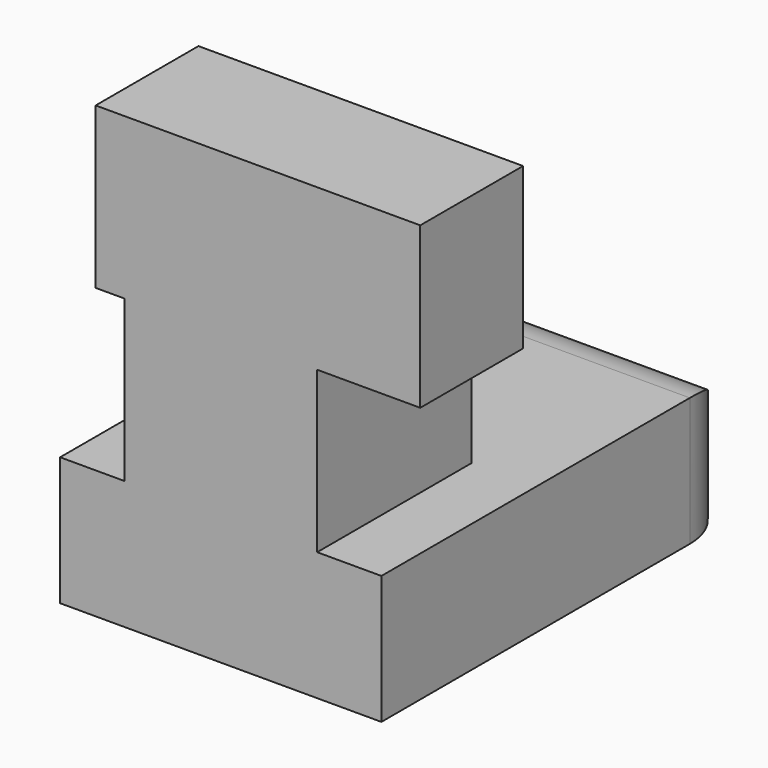
from build123d import *

# Parameters (mm, degrees)
F0_W        = 70
F0_H        = 20
F1_DEPTH    = 25
F2_W        = 30
F2_H        = 30
F3_DEPTH    = 25
F4_R        = 10
F5_W        = 50.5173448473
F5_H        = 20
F6_DEPTH    = 25
F7_T        = 2.5
F7_T3_DEPTH = 35
F7_T5_DEPTH = 35
F7_T7_DEPTH = 25


# Not quite as in the source:
# - a shell that OpenCascade refuses in one call is made with other operations: the cavity is built on its own and cut out


with BuildPart() as f1:
    # F0 (on Right) → F1 (new body, symmetric)
    with BuildSketch(Plane.YZ):
        with Locations((35, 10)):
            Rectangle(F0_W, F0_H)
    extrude(amount=F1_DEPTH, both=True)

    # F2 (on face) → F3 (join)
    with BuildSketch(Plane.XY.offset(20)):
        with Locations((0, 15)):
            Rectangle(F2_W, F2_H)
    extrude(amount=F3_DEPTH)

    # F4
    f4_edges = [f1.edges().sort_by_distance(p)[0] for p in [
        (-25, 70, 10),
        (0, 70, 20),
        (25, 70, 10),
    ]]
    fillet(f4_edges, radius=F4_R)

    # F5 (on face) → F6 (join)
    with BuildSketch(Plane.XY.offset(45)):
        with Locations((5.7856766507, 10)):
            Rectangle(F5_W, F5_H)
    extrude(amount=F6_DEPTH)

    # F7: shell of thickness 2.5, made by hand


with BuildPart() as f7_core1:
    # F7_t2: copy of F1
    add(f1.part)

    # the walls: a layer under each face that stays
    f7_faces = [f7_core1.faces().sort_by_distance(p)[0] for p in [
        (-16.6666666667, 50, 20),
        (25, 30, 10),
        (0, 67.0710678119, 17.0710678119),
        (3.0221745372, 0, 35),
        (-25, 30, 10),
        (15, 15, 32.5),
        (0, 30, 32.5),
        (-15, 15, 32.5),
        (22.0710678119, 67.0710678119, 10),
        (0, 35, 0),
        (0, 70, 5),
        (-22.0710678119, 67.0710678119, 10),
        (23.0221745372, 10, 45),
        (0, 25, 45),
        (-17.2364978865, 10, 45),
        (-19.472995773, 10, 57.5),
        (31.0443490744, 10, 57.5),
        (5.7856766507, 10, 70),
    ]]
    thicken(f7_faces, amount=-F7_T, mode=Mode.SUBTRACT)

    # F7_s4 → F7_t3 (cut)
    with BuildSketch(Plane.XZ.offset(-32.5)):
        Polygon((15.025, 20.025), (15, 17.5), (12.5, 17.5), (12.5, 20), align=None)
        Polygon((-15.025, 20.025), (-15, 17.5), (-12.5, 17.5), (-12.5, 20), align=None)
    extrude(amount=F7_T3_DEPTH, mode=Mode.SUBTRACT)

    # F7_s6 → F7_t5 (cut)
    with BuildSketch(Plane.YZ.offset(-17.5)):
        Polygon((30.025, 20.025), (30, 17.5), (27.5, 17.5), (27.5, 20), align=None)
    extrude(amount=F7_T5_DEPTH, mode=Mode.SUBTRACT)

    # F7_s8 → F7_t7 (cut)
    with BuildSketch(Plane.XZ.offset(-22.5)):
        Polygon((15.025, 44.975), (12.5, 45), (12.5, 47.5), (15, 47.5), align=None)
        Polygon((-15.025, 44.975), (-12.5, 45), (-12.5, 47.5), (-15, 47.5), align=None)
    extrude(amount=F7_T7_DEPTH, mode=Mode.SUBTRACT)


with BuildPart() as f1_1:
    add(f1.part)

    # what is left inside the walls is the cavity
    f7_cavity = [f7_core1.part.solids().sort_by_distance(p)[0] for p in [
        (-7.5, 35, 2.525),
    ]]
    add(f7_cavity, mode=Mode.SUBTRACT)


solid = f1_1.part
